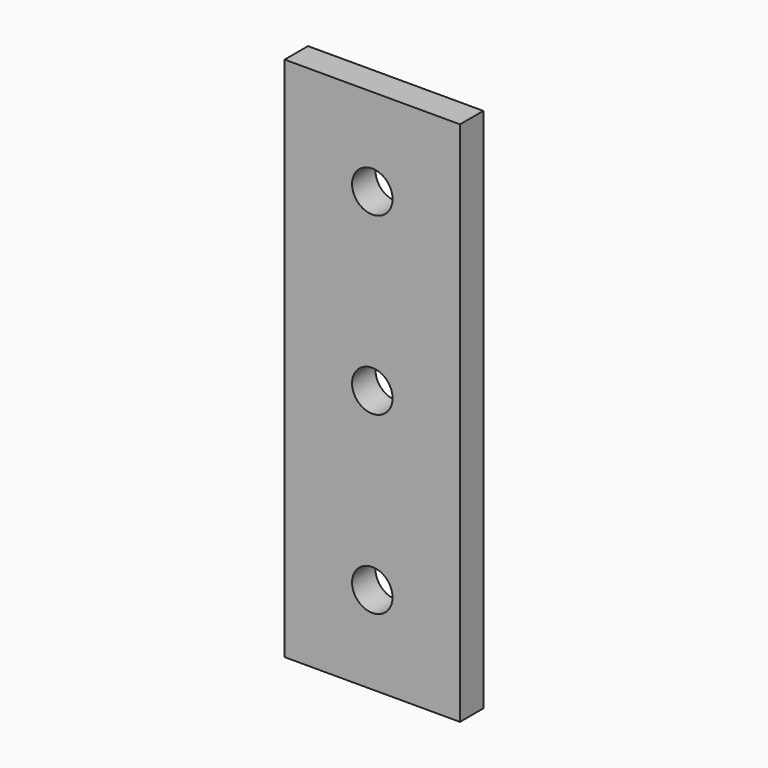
from build123d import *

# Parameters (mm, degrees)
F0_W     = 38.1
F0_H     = 114.3
F1_DEPTH = 6.35
F2_D     = 8.8


# Not quite as in the source:
# - a length typed as a fraction of an inch, garbled in the dataset ("3 / 203.2 mm" for 3/8 in), is restored
# - a feature names something its author has since deleted; it is built from what else it names


with BuildPart() as f1:
    # F0 (on Front) → F1 (new body)
    with BuildSketch(Plane.XZ):
        with Locations((19.05, 57.15)):
            Rectangle(F0_W, F0_H)
    extrude(amount=-F1_DEPTH)

    # F2 (through all)
    with Locations(Plane.XZ):
        with Locations((19.05, 95.25), (19.05, 57.15), (19.05, 19.05)):
            Hole(F2_D / 2)


solid = f1.part
